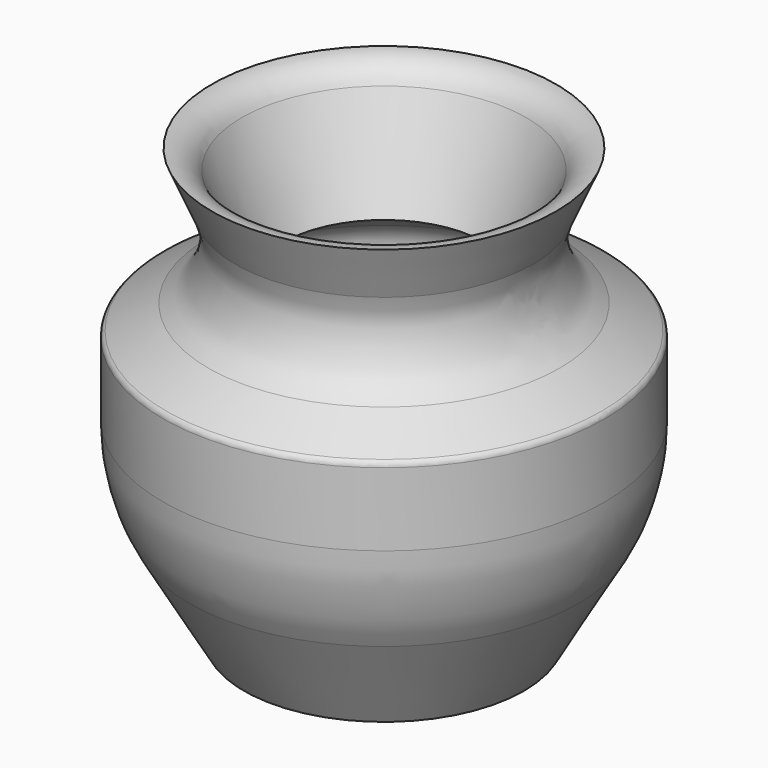
from build123d import *

# Parameters (mm, degrees)
F2_R = 30
F3_R = 10
F4_R = 1


# Not quite as in the source:
# - a fillet or chamfer that OpenCascade refuses, or shapes differently, is made with other operations: its cross-section is extruded or revolved along the edge and cut away or added


with BuildPart() as f1:
    # F0 (on Front) → F1 (revolve)
    with BuildSketch(Plane.XZ):
        with BuildLine():
            Line((0, -21.7408868024), (0, -24.7408868024))
            Line((0, -24.7408868024), (21.4781631635, -24.7408868024))
            Line((21.4781631635, -24.7408868024), (33.8999996632, -3.2256348616))
            Line((33.8999996632, -3.2256348616), (33.8999996632, 16.6180381379))
            Line((33.8999996632, 16.6180381379), (19.2509286784, 25.0756832143))
            Line((19.2509286784, 25.0756832143), (26.4026819505, 41.5839911591))
            Line((26.4026819505, 41.5839911591), (23.6499027339, 42.7765541907))
            Line((23.6499027339, 42.7765541907), (15.4351795785, 23.8146053692))
            Line((15.4351795785, 23.8146053692), (28.3999996632, 16.3293630033))
            ThreePointArc((28.3999996632, 16.3293630033), (30.2301266822, 14.4992359844), (30.8999996632, 11.9992359844))
            Line((30.8999996632, 11.9992359844), (30.8999996632, -1.0820413221))
            ThreePointArc((30.8999996632, -1.0820413221), (30.7296287947, -2.3761365476), (30.2301266822, -3.5820413221))
            Line((30.2301266822, -3.5820413221), (21.1894880289, -19.2408868024))
            ThreePointArc((21.1894880289, -19.2408868024), (19.35936101, -21.0710138213), (16.85936101, -21.7408868024))
            Line((16.85936101, -21.7408868024), (0, -21.7408868024))
        make_face()
    revolve(axis=Axis((0, 0, 6.5311510116), (0, 0, -1)))

    # F2
    f2_edges = [f1.edges().sort_by_distance(p)[0] for p in [
        (-33.9, 0, -3.225635),
    ]]
    fillet(f2_edges, radius=F2_R)

    # F3
    f3_edges = [f1.edges().sort_by_distance(p)[0] for p in [
        (-19.250929, 0, 25.075683),
    ]]
    fillet(f3_edges, radius=F3_R)

    # F4
    f4_edges = [f1.edges().sort_by_distance(p)[0] for p in [
        (-33.9, 0, 16.618038),
    ]]
    fillet(f4_edges, radius=F4_R)

    # F5: fillet of radius 5 on 1 edges, made by hand

    # F5_s1 → F5_t2 (revolve, cut)
    with BuildSketch(Plane.XZ):
        with BuildLine():
            ThreePointArc((26.4026819505, 41.5839911591), (23.6662868758, 40.7598912449), (21.8282326127, 38.5716144801))
            Line((21.8282326127, 38.5716144801), (21.7364733055, 38.6113665812))
            Line((21.7364733055, 38.6113665812), (23.5581434266, 42.8163062918))
            Line((23.5581434266, 42.8163062918), (23.6896548349, 42.8683134979))
            ThreePointArc((23.6896548349, 42.8683134979), (25.0660444432, 42.2720319821), (26.40241163, 41.6839907937))
            Line((26.40241163, 41.6839907937), (26.4026819505, 41.5839911591))
        make_face()
    revolve(axis=Axis((0, 0, 42.7765541907), (0, 0, -1)), mode=Mode.SUBTRACT)


solid = f1.part
